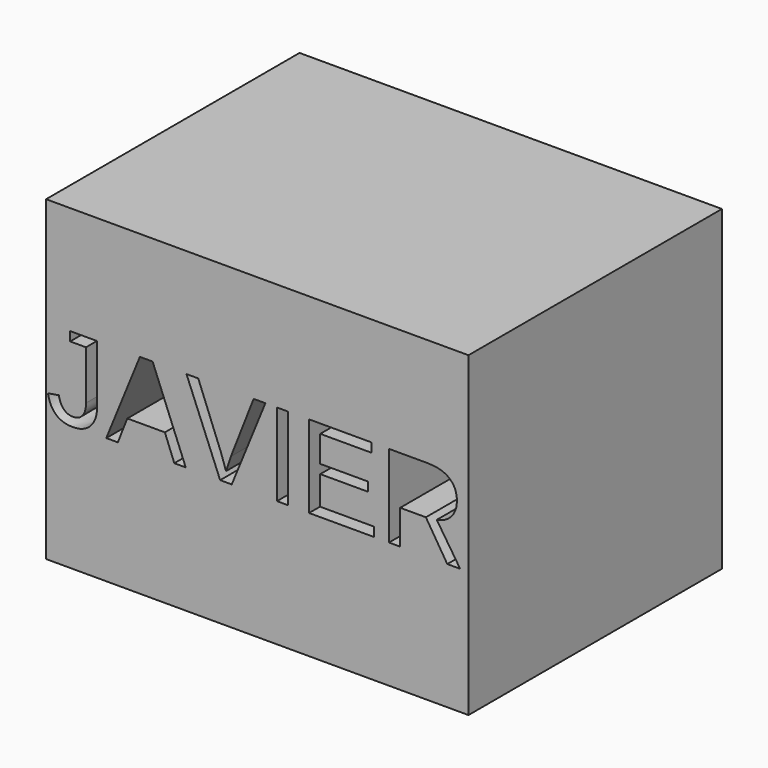
from build123d import *

# Parameters (mm, degrees)
F0_W     = 50.8
F0_H     = 38.1
F0_W_2   = 1.3446661346
F0_H_2   = 9.9171942893
F1_DEPTH = 12.7
F2_DEPTH = 25.4


with BuildPart() as f1:
    # F0 (on Front) → F1 (new body, symmetric)
    with BuildSketch(Plane.XZ):
        with Locations((-36.0804582015, 47.4701705396)):
            Rectangle(F0_W, F0_H)
        with BuildLine():
            add(Edge.make_bspline(
                [(-56.1243173839, 44.267506293), (-56.9058904973, 43.4397595518), (-58.2640708644, 43.4397595518)],
                knots=[0, 0, 0, 1, 1, 1], degree=2))
            add(Edge.make_bspline(
                [(-58.2640708644, 43.4397595518), (-60.7844752273, 43.4397595518), (-61.255220993, 46.0457540539)],
                knots=[0, 0, 0, 1, 1, 1], degree=2))
            Line((-61.255220993, 46.0457540539), (-59.9398356955, 46.2642341461))
            add(Edge.make_bspline(
                [(-59.9398356955, 46.2642341461), (-59.8114504867, 45.4466230794), (-59.368859372, 44.9893915462)],
                knots=[0, 0, 0, 1, 1, 1], degree=2))
            add(Edge.make_bspline(
                [(-59.368859372, 44.9893915462), (-58.9262682573, 44.5321600129), (-58.2573137482, 44.5321600129)],
                knots=[0, 0, 0, 1, 1, 1], degree=2))
            add(Edge.make_bspline(
                [(-58.2573137482, 44.5321600129), (-57.5252928206, 44.5321600129), (-57.1029730547, 45.0355651739)],
                knots=[0, 0, 0, 1, 1, 1], degree=2))
            add(Edge.make_bspline(
                [(-57.1029730547, 45.0355651739), (-56.6806532888, 45.5389703348), (-56.6806532888, 46.5097427034)],
                knots=[0, 0, 0, 1, 1, 1], degree=2))
            Line((-56.6806532888, 46.5097427034), (-56.6806532888, 52.4019480771))
            Line((-56.6806532888, 52.4019480771), (-58.5884124446, 52.4019480771))
            Line((-58.5884124446, 52.4019480771), (-58.5884124446, 53.4988532824))
            Line((-58.5884124446, 53.4988532824), (-55.3427442705, 53.4988532824))
            Line((-55.3427442705, 53.4988532824), (-55.3427442705, 46.5390235405))
            add(Edge.make_bspline(
                [(-55.3427442705, 46.5390235405), (-55.3427442705, 45.0952530341), (-56.1243173839, 44.267506293)],
                knots=[0, 0, 0, 1, 1, 1], degree=2))
        make_face(mode=Mode.SUBTRACT)
        Polygon((-44.6867719374, 43.5816589932), (-46.058466537, 43.5816589932), (-47.1914096957, 46.4827142384), (-51.7096680977, 46.4827142384), (-52.8516207447, 43.5816589932), (-54.2435866931, 43.5816589932), (-50.1983264288, 53.4988532824), (-48.6689657833, 53.4988532824), align=None, mode=Mode.SUBTRACT)
        Polygon((-35.1051810888, 53.4988532824), (-39.1526937251, 43.5816589932), (-40.5469120456, 43.5816589932), (-44.5944246819, 53.4988532824), (-43.1799350127, 53.4988532824), (-40.4342934413, 46.5164998196), (-39.841919583, 44.7641543377), (-39.2517980968, 46.5164998196), (-36.519670758, 53.4988532824), align=None, mode=Mode.SUBTRACT)
        with Locations((-33.038629701, 48.5402561378)):
            Rectangle(F0_W_2, F0_H_2, mode=Mode.SUBTRACT)
        Polygon((-22.0414229971, 43.5816589932), (-29.8549017592, 43.5816589932), (-29.8549017592, 53.4988532824), (-22.3297266239, 53.4988532824), (-22.3297266239, 52.4019480771), (-28.5102356245, 52.4019480771), (-28.5102356245, 49.2193463214), (-22.7531725759, 49.2193463214), (-22.7531725759, 48.1359553486), (-28.5102356245, 48.1359553486), (-28.5102356245, 44.6808165705), (-22.0414229971, 44.6808165705), align=None, mode=Mode.SUBTRACT)
        with BuildLine():
            Line((-11.6805114071, 43.5816589932), (-13.2278910293, 43.5816589932))
            Line((-13.2278910293, 43.5816589932), (-15.8046046943, 47.6989951641))
            Line((-15.8046046943, 47.6989951641), (-18.8948591946, 47.6989951641))
            Line((-18.8948591946, 47.6989951641), (-18.8948591946, 43.5816589932))
            Line((-18.8948591946, 43.5816589932), (-20.2395253293, 43.5816589932))
            Line((-20.2395253293, 43.5816589932), (-20.2395253293, 53.4988532824))
            Line((-20.2395253293, 53.4988532824), (-15.5726103696, 53.4988532824))
            add(Edge.make_bspline(
                [(-15.5726103696, 53.4988532824), (-13.8968455385, 53.4988532824), (-12.9857610302, 52.7499395642)],
                knots=[0, 0, 0, 1, 1, 1], degree=2))
            add(Edge.make_bspline(
                [(-12.9857610302, 52.7499395642), (-12.0746765219, 52.0010258461), (-12.0746765219, 50.6631168277)],
                knots=[0, 0, 0, 1, 1, 1], degree=2))
            add(Edge.make_bspline(
                [(-12.0746765219, 50.6631168277), (-12.0746765219, 49.5572021341), (-12.7188549382, 48.8037836717)],
                knots=[0, 0, 0, 1, 1, 1], degree=2))
            add(Edge.make_bspline(
                [(-12.7188549382, 48.8037836717), (-13.3630333544, 48.0503652094), (-14.4959765131, 47.854408838)],
                knots=[0, 0, 0, 1, 1, 1], degree=2))
            Line((-14.4959765131, 47.854408838), (-11.6805114071, 43.5816589932))
        make_face(mode=Mode.SUBTRACT)
    extrude(amount=F1_DEPTH, both=True)

    # F0 (on Front) → F2 (join)
    with BuildSketch(Plane.XZ):
        with Locations((-36.0804582015, 47.4701705396)):
            Rectangle(F0_W, F0_H)
        with BuildLine():
            add(Edge.make_bspline(
                [(-56.1243173839, 44.267506293), (-56.9058904973, 43.4397595518), (-58.2640708644, 43.4397595518)],
                knots=[0, 0, 0, 1, 1, 1], degree=2))
            add(Edge.make_bspline(
                [(-58.2640708644, 43.4397595518), (-60.7844752273, 43.4397595518), (-61.255220993, 46.0457540539)],
                knots=[0, 0, 0, 1, 1, 1], degree=2))
            Line((-61.255220993, 46.0457540539), (-59.9398356955, 46.2642341461))
            add(Edge.make_bspline(
                [(-59.9398356955, 46.2642341461), (-59.8114504867, 45.4466230794), (-59.368859372, 44.9893915462)],
                knots=[0, 0, 0, 1, 1, 1], degree=2))
            add(Edge.make_bspline(
                [(-59.368859372, 44.9893915462), (-58.9262682573, 44.5321600129), (-58.2573137482, 44.5321600129)],
                knots=[0, 0, 0, 1, 1, 1], degree=2))
            add(Edge.make_bspline(
                [(-58.2573137482, 44.5321600129), (-57.5252928206, 44.5321600129), (-57.1029730547, 45.0355651739)],
                knots=[0, 0, 0, 1, 1, 1], degree=2))
            add(Edge.make_bspline(
                [(-57.1029730547, 45.0355651739), (-56.6806532888, 45.5389703348), (-56.6806532888, 46.5097427034)],
                knots=[0, 0, 0, 1, 1, 1], degree=2))
            Line((-56.6806532888, 46.5097427034), (-56.6806532888, 52.4019480771))
            Line((-56.6806532888, 52.4019480771), (-58.5884124446, 52.4019480771))
            Line((-58.5884124446, 52.4019480771), (-58.5884124446, 53.4988532824))
            Line((-58.5884124446, 53.4988532824), (-55.3427442705, 53.4988532824))
            Line((-55.3427442705, 53.4988532824), (-55.3427442705, 46.5390235405))
            add(Edge.make_bspline(
                [(-55.3427442705, 46.5390235405), (-55.3427442705, 45.0952530341), (-56.1243173839, 44.267506293)],
                knots=[0, 0, 0, 1, 1, 1], degree=2))
        make_face(mode=Mode.SUBTRACT)
        Polygon((-44.6867719374, 43.5816589932), (-46.058466537, 43.5816589932), (-47.1914096957, 46.4827142384), (-51.7096680977, 46.4827142384), (-52.8516207447, 43.5816589932), (-54.2435866931, 43.5816589932), (-50.1983264288, 53.4988532824), (-48.6689657833, 53.4988532824), align=None, mode=Mode.SUBTRACT)
        Polygon((-35.1051810888, 53.4988532824), (-39.1526937251, 43.5816589932), (-40.5469120456, 43.5816589932), (-44.5944246819, 53.4988532824), (-43.1799350127, 53.4988532824), (-40.4342934413, 46.5164998196), (-39.841919583, 44.7641543377), (-39.2517980968, 46.5164998196), (-36.519670758, 53.4988532824), align=None, mode=Mode.SUBTRACT)
        with Locations((-33.038629701, 48.5402561378)):
            Rectangle(F0_W_2, F0_H_2, mode=Mode.SUBTRACT)
        Polygon((-22.0414229971, 43.5816589932), (-29.8549017592, 43.5816589932), (-29.8549017592, 53.4988532824), (-22.3297266239, 53.4988532824), (-22.3297266239, 52.4019480771), (-28.5102356245, 52.4019480771), (-28.5102356245, 49.2193463214), (-22.7531725759, 49.2193463214), (-22.7531725759, 48.1359553486), (-28.5102356245, 48.1359553486), (-28.5102356245, 44.6808165705), (-22.0414229971, 44.6808165705), align=None, mode=Mode.SUBTRACT)
        with BuildLine():
            Line((-11.6805114071, 43.5816589932), (-13.2278910293, 43.5816589932))
            Line((-13.2278910293, 43.5816589932), (-15.8046046943, 47.6989951641))
            Line((-15.8046046943, 47.6989951641), (-18.8948591946, 47.6989951641))
            Line((-18.8948591946, 47.6989951641), (-18.8948591946, 43.5816589932))
            Line((-18.8948591946, 43.5816589932), (-20.2395253293, 43.5816589932))
            Line((-20.2395253293, 43.5816589932), (-20.2395253293, 53.4988532824))
            Line((-20.2395253293, 53.4988532824), (-15.5726103696, 53.4988532824))
            add(Edge.make_bspline(
                [(-15.5726103696, 53.4988532824), (-13.8968455385, 53.4988532824), (-12.9857610302, 52.7499395642)],
                knots=[0, 0, 0, 1, 1, 1], degree=2))
            add(Edge.make_bspline(
                [(-12.9857610302, 52.7499395642), (-12.0746765219, 52.0010258461), (-12.0746765219, 50.6631168277)],
                knots=[0, 0, 0, 1, 1, 1], degree=2))
            add(Edge.make_bspline(
                [(-12.0746765219, 50.6631168277), (-12.0746765219, 49.5572021341), (-12.7188549382, 48.8037836717)],
                knots=[0, 0, 0, 1, 1, 1], degree=2))
            add(Edge.make_bspline(
                [(-12.7188549382, 48.8037836717), (-13.3630333544, 48.0503652094), (-14.4959765131, 47.854408838)],
                knots=[0, 0, 0, 1, 1, 1], degree=2))
            Line((-14.4959765131, 47.854408838), (-11.6805114071, 43.5816589932))
        make_face(mode=Mode.SUBTRACT)
    extrude(amount=F2_DEPTH)


solid = f1.part
